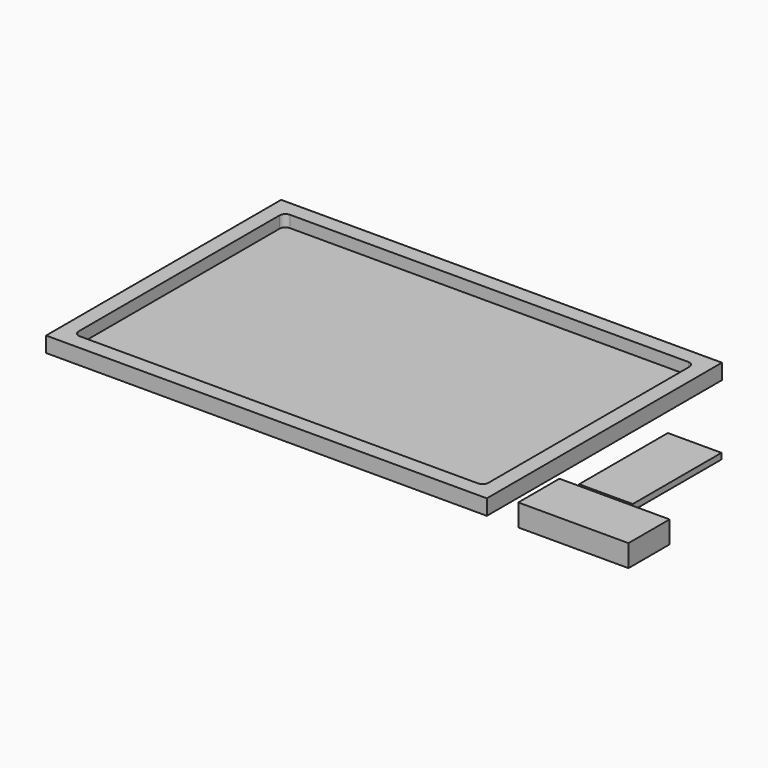
from build123d import *

# Parameters (mm, degrees)
F1_W     = 600
F1_H     = 400
F2_DEPTH = 21
F3_DEPTH = 5
F1_W_2   = 150
F1_H_2   = 70
F4_DEPTH = 30
F1_W_3   = 73
F1_H_3   = 151
F5_DEPTH = 8


with BuildPart() as f2:
    # F1 (on Top) → F2 (new body)
    with BuildSketch(Plane.XY):
        with Locations((300, 200)):
            Rectangle(F1_W, F1_H)
        with BuildLine():
            ThreePointArc((21, 371), (23.3431457505, 376.6568542495), (29, 379))
            Line((29, 379), (571, 379))
            ThreePointArc((571, 379), (576.6568542495, 376.6568542495), (579, 371))
            Line((579, 371), (579, 29))
            ThreePointArc((579, 29), (576.6568542495, 23.3431457505), (571, 21))
            Line((571, 21), (29, 21))
            ThreePointArc((29, 21), (23.3431457505, 23.3431457505), (21, 29))
            Line((21, 29), (21, 371))
        make_face(mode=Mode.SUBTRACT)
    extrude(amount=F2_DEPTH)

    # F1 (on Top) → F3 (join)
    with BuildSketch(Plane.XY):
        with BuildLine():
            Line((571, 379), (29, 379))
            ThreePointArc((29, 379), (23.3431457505, 376.6568542495), (21, 371))
            Line((21, 371), (21, 29))
            ThreePointArc((21, 29), (23.3431457505, 23.3431457505), (29, 21))
            Line((29, 21), (571, 21))
            ThreePointArc((571, 21), (576.6568542495, 23.3431457505), (579, 29))
            Line((579, 29), (579, 371))
            ThreePointArc((579, 371), (576.6568542495, 376.6568542495), (571, 379))
        make_face()
    extrude(amount=F3_DEPTH)


with BuildPart() as f4:
    # F1 (on Top) → F4 (new body)
    with BuildSketch(Plane.XY):
        with Locations((717.7889823914, 35)):
            Rectangle(F1_W_2, F1_H_2)
    extrude(amount=F4_DEPTH)


with BuildPart() as f5:
    # F1 (on Top) → F5 (new body)
    with BuildSketch(Plane.XY):
        with Locations((677.1741738319, 181.6440706253)):
            Rectangle(F1_W_3, F1_H_3)
    extrude(amount=F5_DEPTH)


solid = Compound([f2.part, f4.part, f5.part])
